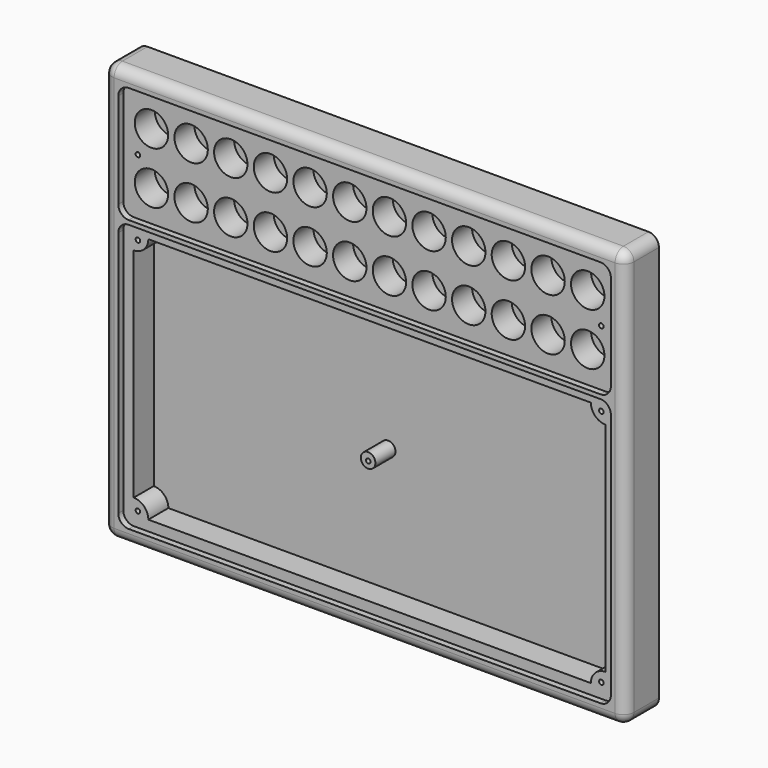
from build123d import *

# Parameters (mm, degrees)
F1_DEPTH = 20
F2_R     = 5
F5_DEPTH = 3
F6_R     = 8
F6_R_2   = 3.5
F7_DEPTH = 15
F8_R     = 1.1
F9_DEPTH = 10


with BuildPart() as f1:
    # F0 (on Front) → F1 (new body)
    with BuildSketch(Plane.XZ):
        with BuildLine():
            ThreePointArc((0, 5), (1.4644660941, 1.4644660941), (5, 0))
            Line((5, 0), (245, 0))
            ThreePointArc((245, 0), (248.5355339059, 1.4644660941), (250, 5))
            Line((250, 5), (250, 195))
            ThreePointArc((250, 195), (248.5355339059, 198.5355339059), (245, 200))
            Line((245, 200), (5, 200))
            ThreePointArc((5, 200), (1.4644660941, 198.5355339059), (0, 195))
            Line((0, 195), (0, 5))
        make_face()
    extrude(amount=-F1_DEPTH)

    # F2
    f2_edges = [f1.edges().sort_by_distance(p)[0] for p in [
        (0, 0, 100),
        (1.464466, 0, 1.464466),
        (125, 0, 0),
        (248.535534, 0, 1.464466),
        (250, 0, 100),
        (248.535534, 0, 198.535534),
        (125, 0, 200),
        (1.464466, 0, 198.535534),
    ]]
    fillet(f2_edges, radius=F2_R)

    # F4 (on face) → F5 (cut)
    with BuildSketch(Plane.XZ):
        with BuildLine():
            ThreePointArc((243, 188), (241.5355339059, 191.5355339059), (238, 193))
            Line((238, 193), (12, 193))
            ThreePointArc((12, 193), (8.4644660941, 191.5355339059), (7, 188))
            Line((7, 188), (7, 142.2841556072))
            ThreePointArc((7, 142.2841556072), (8.4644660941, 138.7486217013), (12, 137.2841556072))
            Line((12, 137.2841556072), (238, 137.2841556072))
            ThreePointArc((238, 137.2841556072), (241.5355339059, 138.7486217013), (243, 142.2841556072))
            Line((243, 142.2841556072), (243, 188))
        make_face()
        with BuildLine():
            ThreePointArc((238, 7), (241.5355339059, 8.4644660941), (243, 12))
            Line((243, 12), (243, 130.2841556072))
            ThreePointArc((243, 130.2841556072), (241.5355339059, 133.8196895132), (238, 135.2841556072))
            Line((238, 135.2841556072), (12, 135.2841556072))
            ThreePointArc((12, 135.2841556072), (8.4644660941, 133.8196895132), (7, 130.2841556072))
            Line((7, 130.2841556072), (7, 12))
            ThreePointArc((7, 12), (8.4644660941, 8.4644660941), (12, 7))
            Line((12, 7), (238, 7))
        make_face()
    extrude(amount=-F5_DEPTH, mode=Mode.SUBTRACT)

    # F6 (on face) → F7 (cut)
    with BuildSketch(Plane.XZ):
        with Locations((20.5, 152.2841556072)):
            Circle(F6_R)
        with Locations((20.5, 177.2841556072)):
            Circle(F6_R)
        with Locations((39.5, 152.2841556072)):
            Circle(F6_R)
        with Locations((39.5, 177.2841556072)):
            Circle(F6_R)
        with Locations((58.5, 152.2841556072)):
            Circle(F6_R)
        with Locations((58.5, 177.2841556072)):
            Circle(F6_R)
        with Locations((77.5, 152.2841556072)):
            Circle(F6_R)
        with Locations((77.5, 177.2841556072)):
            Circle(F6_R)
        with Locations((96.5, 152.2841556072)):
            Circle(F6_R)
        with Locations((96.5, 177.2841556072)):
            Circle(F6_R)
        with Locations((115.5, 152.2841556072)):
            Circle(F6_R)
        with Locations((115.5, 177.2841556072)):
            Circle(F6_R)
        with Locations((134.5, 152.2841556072)):
            Circle(F6_R)
        with Locations((134.5, 177.2841556072)):
            Circle(F6_R)
        with Locations((153.5, 152.2841556072)):
            Circle(F6_R)
        with Locations((153.5, 177.2841556072)):
            Circle(F6_R)
        with Locations((172.5, 152.2841556072)):
            Circle(F6_R)
        with Locations((172.5, 177.2841556072)):
            Circle(F6_R)
        with Locations((191.5, 152.2841556072)):
            Circle(F6_R)
        with Locations((191.5, 177.2841556072)):
            Circle(F6_R)
        with Locations((210.5, 152.2841556072)):
            Circle(F6_R)
        with Locations((210.5, 177.2841556072)):
            Circle(F6_R)
        with Locations((229.5, 152.2841556072)):
            Circle(F6_R)
        with Locations((229.5, 177.2841556072)):
            Circle(F6_R)
        with BuildLine():
            Line((231, 130.2841556072), (19, 130.2841556072))
            ThreePointArc((19, 130.2841556072), (16.9497474683, 125.3344081389), (12, 123.2841556072))
            Line((12, 123.2841556072), (12, 19))
            ThreePointArc((12, 19), (16.9497474683, 16.9497474683), (19, 12))
            Line((19, 12), (231, 12))
            ThreePointArc((231, 12), (233.0502525317, 16.9497474683), (238, 19))
            Line((238, 19), (238, 123.2841556072))
            ThreePointArc((238, 123.2841556072), (233.0502525317, 125.3344081389), (231, 130.2841556072))
        make_face()
        with Locations((124.2906078696, 71.2240189314)):
            Circle(F6_R_2, mode=Mode.SUBTRACT)
    extrude(amount=-F7_DEPTH, mode=Mode.SUBTRACT)

    # F8 (on face) → F9 (cut)
    with BuildSketch(Plane.XZ):
        with Locations((14, 128.2841556072)):
            Circle(F8_R)
        with Locations((14, 14)):
            Circle(F8_R)
        with Locations((124.4, 71)):
            Circle(F8_R)
        with Locations((236, 14)):
            Circle(F8_R)
        with Locations((236, 128.2841556072)):
            Circle(F8_R)
        with Locations((236, 164.2841556072)):
            Circle(F8_R)
        with Locations((14, 164.2841556072)):
            Circle(F8_R)
    extrude(amount=-F9_DEPTH, mode=Mode.SUBTRACT)


solid = f1.part
